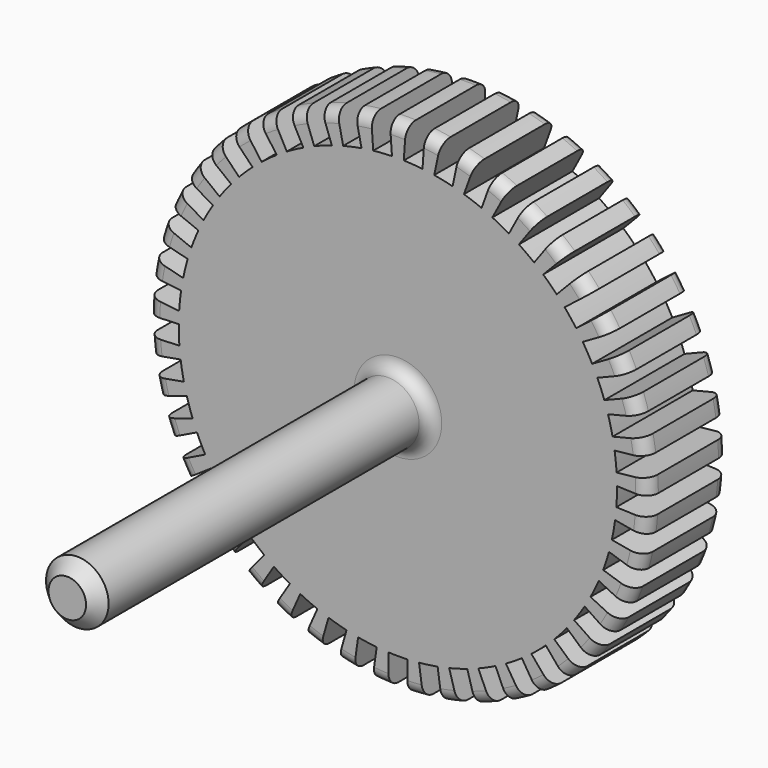
from build123d import *

# Parameters (mm, degrees)
F0_R            = 200
F0_R_2          = 175
F0_R_3          = 25
F1_DEPTH        = 80
F2_DEPTH        = 410
F3_R            = 10
F4_SIZE         = 10
F6_DEPTH        = 410.001
F6_COPIES_COUNT = 45


# Not quite as in the source:
# - a pattern or mirror of a feature is missing from the dataset's text; its kind, count and spacing are read off the source's solid


with BuildPart() as f1:
    # F0 (on Front) → F1 (new body)
    with BuildSketch(Plane.XZ):
        Circle(F0_R)
        Circle(F0_R_2, mode=Mode.SUBTRACT)
        Circle(F0_R_2)
        Circle(F0_R_3, mode=Mode.SUBTRACT)
    extrude(amount=F1_DEPTH)

    # F0 (on Front) → F2 (join)
    with BuildSketch(Plane.XZ):
        Circle(F0_R_3)
    extrude(amount=F2_DEPTH)

    # F3
    f3_edges = [f1.edges().sort_by_distance(p)[0] for p in [
        (-200, 0, 0),
        (-200, -80, 0),
        (-25, -80, 0),
    ]]
    fillet(f3_edges, radius=F3_R)

    # F4
    f4_edges = [f1.edges().sort_by_distance(p)[0] for p in [
        (-25, -410, 0),
    ]]
    chamfer(f4_edges, length=F4_SIZE)

    # F5 (on Front) → F6 (cut, through all)
    with BuildSketch(Plane.XZ):
        with BuildLine():
            ThreePointArc((7.5, -174.8392118491), (0, -175), (-7.5, -174.8392118491))
            Line((-7.5, -174.8392118491), (-7.5, -213.8746801315))
            Line((-7.5, -213.8746801315), (7.5, -213.8746801315))
            Line((7.5, -213.8746801315), (7.5, -174.8392118491))
        make_face()
    f6 = extrude(amount=F6_DEPTH, mode=Mode.SUBTRACT)

    # F6_copies: F6 ×45 about axis
    f6_copies_axis = Axis((0, 0, 0), (0, 1, 0))
    for i in range(1, F6_COPIES_COUNT):
        add(f6.rotate(f6_copies_axis, i * 360 / F6_COPIES_COUNT), mode=Mode.SUBTRACT)


solid = f1.part
